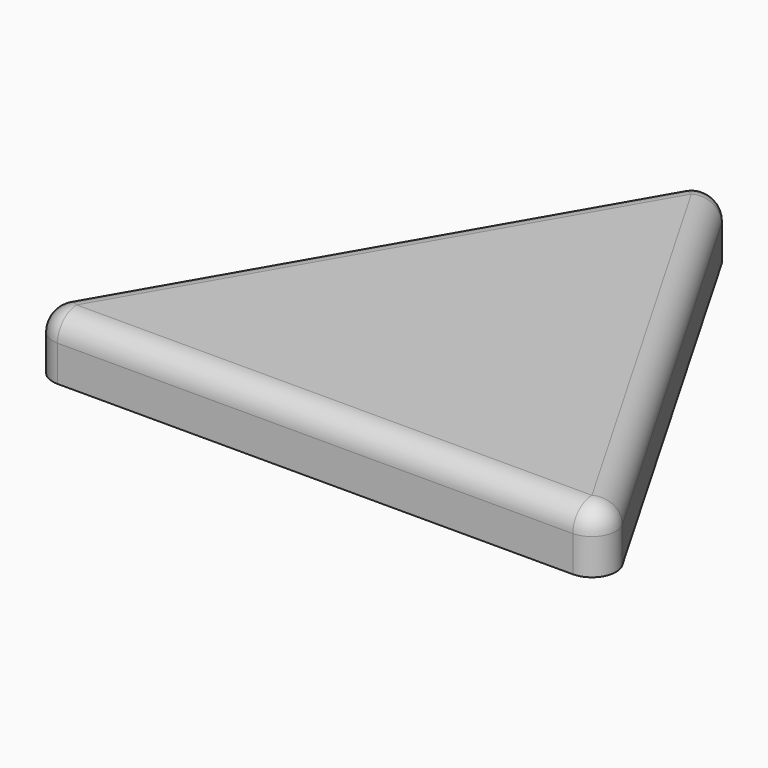
from build123d import *

# Parameters (mm, degrees)
F1_DEPTH     = 25
F2_R         = 10
F3_T1_DEPTH  = 257.6794919243
F3_T3_DEPTH  = 58.3012701892
F3_T8_DEPTH  = 10
F4_T1_DEPTH  = 215.3589838486
F4_T3_DEPTH  = 58.3012701892
F4_T8_DEPTH  = 10
F4_T14_DEPTH = 10


# Not quite as in the source:
# - a fillet or chamfer that OpenCascade refuses, or shapes differently, is made with other operations: its cross-section is extruded or revolved along the edge and cut away or added


with BuildPart() as f1:
    # F0 (on Top) → F1 (new body)
    with BuildSketch(Plane.XY):
        Polygon((125, -216.5063509461), (0, 0), (-125, -216.5063509461), align=None)
    extrude(amount=F1_DEPTH)

    # F2
    f2_edges = [f1.edges().sort_by_distance(p)[0] for p in [
        (0, -216.506351, 25),
    ]]
    fillet(f2_edges, radius=F2_R)

    # F3: fillet of radius 10 on 1 edges, made by hand

    # F3_s2 → F3_t1 (cut)
    with BuildSketch(Plane(origin=(116.3397459622, -201.5063509461, 0), x_dir=(0, 0, 1), z_dir=(-0.5, 0.8660254038, 0))):
        with BuildLine():
            ThreePointArc((15, 0), (22.0710678119, -2.9289321881), (25, -10))
            Line((25, -10), (25, 0))
            Line((25, 0), (15, 0))
        make_face()
    extrude(amount=F3_T1_DEPTH, mode=Mode.SUBTRACT)

    # F3_s4 → F3_t3 (cut)
    with BuildSketch(Plane.XY.offset(-43.3012701892)):
        with BuildLine():
            ThreePointArc((116.3397459622, -201.5063509461), (116.3397459622, -211.5063509461), (107.6794919243, -216.5063509461))
            Line((107.6794919243, -216.5063509461), (125, -216.5063509461))
            Line((125, -216.5063509461), (116.3397459622, -201.5063509461))
        make_face()
    extrude(amount=F3_T3_DEPTH, mode=Mode.SUBTRACT)


with BuildPart() as f3_tool6:
    # F3_s7 → F3_t8 (new body)
    with BuildSketch(Plane.XY.offset(15)):
        Polygon((107.6794919243, -206.5063509461), (116.3397459622, -201.5063509461), (125, -216.5063509461), (107.6794919243, -216.5063509461), align=None)
    extrude(amount=F3_T8_DEPTH)

    # F3_s9 → F3_t10 (revolve, cut)
    with BuildSketch(Plane(origin=(107.6794919243, -206.5063509461, 15), x_dir=(-0.8660254038, 0.5, 0), z_dir=(0.5, 0.8660254038, 0))):
        with BuildLine():
            ThreePointArc((0, -10), (10, 0), (0, 10))
            Line((0, 10), (0, -10))
        make_face()
    revolve(axis=Axis((107.6794919243, -206.5063509461, 15), (0, 0, 1)), mode=Mode.SUBTRACT)


with BuildPart() as f1_1:
    add(f1.part)

    # F3_t5: cut F3_tool6
    add(f3_tool6.part, mode=Mode.SUBTRACT)

    # F4: fillet of radius 10 on 3 edges, made by hand

    # F4_s2 → F4_t1 (cut)
    with BuildSketch(Plane(origin=(-8.6602540378, -15, 0), x_dir=(0, 0, 1), z_dir=(-0.5, -0.8660254038, 0))):
        with BuildLine():
            ThreePointArc((15, 0), (22.0710678119, -2.9289321881), (25, -10))
            Line((25, -10), (25, 0))
            Line((25, 0), (15, 0))
        make_face()
    extrude(amount=F4_T1_DEPTH, mode=Mode.SUBTRACT)

    # F4_s4 → F4_t3 (cut)
    with BuildSketch(Plane.XY.offset(-43.3012701892)):
        with BuildLine():
            ThreePointArc((8.6602540378, -15), (0, -10), (-8.6602540378, -15))
            Line((-8.6602540378, -15), (0, 0))
            Line((0, 0), (8.6602540378, -15))
        make_face()
        with BuildLine():
            ThreePointArc((-116.3397459622, -201.5063509461), (-116.3397459622, -211.5063509461), (-107.6794919243, -216.5063509461))
            Line((-107.6794919243, -216.5063509461), (-125, -216.5063509461))
            Line((-125, -216.5063509461), (-116.3397459622, -201.5063509461))
        make_face()
    extrude(amount=F4_T3_DEPTH, mode=Mode.SUBTRACT)


with BuildPart() as f4_tool6:
    # F4_s7 → F4_t8 (new body)
    with BuildSketch(Plane.XY.offset(15)):
        Polygon((-107.6794919243, -206.5063509461), (-116.3397459622, -201.5063509461), (-125, -216.5063509461), (-107.6794919243, -216.5063509461), align=None)
    extrude(amount=F4_T8_DEPTH)

    # F4_s9 → F4_t10 (revolve, cut)
    with BuildSketch(Plane(origin=(-107.6794919243, -206.5063509461, 15), x_dir=(0.8660254038, 0.5, 0), z_dir=(0.5, -0.8660254038, 0))):
        with BuildLine():
            ThreePointArc((0, -10), (10, 0), (0, 10))
            Line((0, 10), (0, -10))
        make_face()
    revolve(axis=Axis((-107.6794919243, -206.5063509461, 15), (0, 0, 1)), mode=Mode.SUBTRACT)


with BuildPart() as f1_2:
    add(f1_1.part)

    # F4_t5: cut F4_tool6
    add(f4_tool6.part, mode=Mode.SUBTRACT)


with BuildPart() as f4_tool12:
    # F4_s13 → F4_t14 (new body)
    with BuildSketch(Plane.XY.offset(15)):
        Polygon((0, -20), (8.6602540378, -15), (0, 0), (-8.6602540378, -15), align=None)
    extrude(amount=F4_T14_DEPTH)

    # F4_s15 → F4_t16 (revolve, cut)
    with BuildSketch(Plane(origin=(0, -20, 15), x_dir=(0, -1, 0), z_dir=(-1, 0, 0))):
        with BuildLine():
            ThreePointArc((0, -10), (10, 0), (0, 10))
            Line((0, 10), (0, -10))
        make_face()
    revolve(axis=Axis((0, -20, 15), (0, 0, 1)), mode=Mode.SUBTRACT)


with BuildPart() as f1_3:
    add(f1_2.part)

    # F4_t11: cut F4_tool12
    add(f4_tool12.part, mode=Mode.SUBTRACT)


solid = f1_3.part
